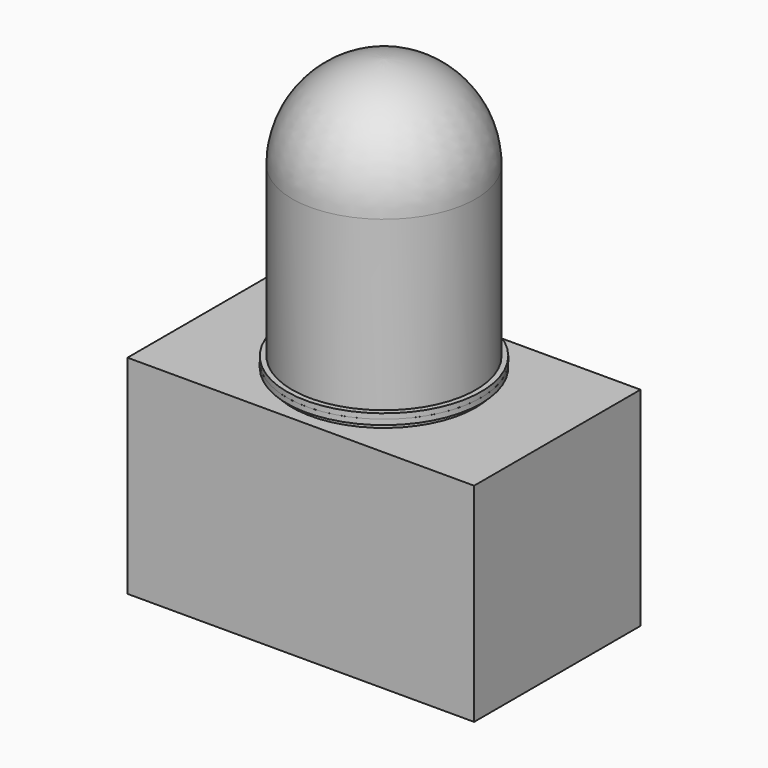
from build123d import *

# Parameters (mm, degrees)
F0_W      = 3
F0_H      = 3
F2_R      = 56
F2_R_2    = 50
F3_DEPTH  = 3
F4_R      = 53
F4_R_2    = 50
F5_DEPTH  = 3
F6_W      = 200
F6_H      = 120
F7_DEPTH  = 120
F8_T      = 3
F9_R      = 50
F10_DEPTH = 4


# Not quite as in the source:
# - a shell that OpenCascade refuses in one call is made with other operations: the cavity is built on its own and cut out


with BuildPart() as f1:
    # F0 (on Front) → F1 (revolve)
    with BuildSketch(Plane.XZ):
        with Locations((-54.5, 1.5)):
            Rectangle(F0_W, F0_H)
        Polygon((-53, 3), (-53, 0), (-50, 0), (-50, 100), (-53, 100), align=None)
        with BuildLine():
            Line((-53, 100), (-50, 100))
            ThreePointArc((-50, 100), (-35.4201251719, 135.7429342759), (0, 151.0904042125))
            Line((0, 151.0904042125), (0, 154.0904042125))
            ThreePointArc((0, 154.0904042125), (-37.5415211912, 137.8641381384), (-53, 100))
        make_face()
    revolve(axis=Axis((0, 0, 55.2105903625), (0, 0, 1)))


with BuildPart() as f3:
    # F2 (on face) → F3 (new body)
    with BuildSketch(Plane(origin=(0, 0, 0), x_dir=(1, 0, 0), z_dir=(0, 0, -1))):
        Circle(F2_R)
        Circle(F2_R_2, mode=Mode.SUBTRACT)
    extrude(amount=F3_DEPTH)

    # F4 (on face) → F5 (join)
    with BuildSketch(Plane(origin=(0, 0, -3), x_dir=(1, 0, 0), z_dir=(0, 0, -1))):
        Circle(F4_R)
        Circle(F4_R_2, mode=Mode.SUBTRACT)
    extrude(amount=F5_DEPTH)

    # F6 (on face) → F7 (join)
    with BuildSketch(Plane(origin=(0, 0, -6), x_dir=(1, 0, 0), z_dir=(0, 0, -1))):
        Rectangle(F6_W, F6_H)
    extrude(amount=F7_DEPTH)

    # F8: shell of thickness 3, made by hand


with BuildPart() as f8_core1:
    # F8_t2: copy of F3
    add(f3.part)

    # the walls: a layer under each face that stays
    f8_faces = [f8_core1.faces().sort_by_distance(p)[0] for p in [
        (0, -60, -66),
        (100, 0, -66),
        (-100, 0, -66),
        (-66.6666666667, 40, -6),
        (0, 60, -66),
        (-53, 0, -4.5),
        (-52.2666666667, 14.9333333333, -3),
        (-56, 0, -1.5),
        (-37.3333333333, 37.3333333333, 0),
        (-50, 0, -3),
        (0, 0, -6),
    ]]
    thicken(f8_faces, amount=-F8_T, mode=Mode.SUBTRACT)

    # F8_s3 → F8_t4 (revolve, cut)
    with BuildSketch(Plane.XZ):
        Polygon((53.03, -5.97), (53, -9), (50, -9), (50, -6), align=None)
    revolve(axis=Axis((0, 0, -6), (0, 0, -1)), mode=Mode.SUBTRACT)

    # F8_s5 → F8_t6 (revolve, cut)
    with BuildSketch(Plane.XZ):
        Polygon((53.03, -3.03), (50, -3), (50, 0), (53, 0), align=None)
    revolve(axis=Axis((0, 0, -3), (0, 0, -1)), mode=Mode.SUBTRACT)

    # F8_s7 → F8_t8 (revolve, cut)
    with BuildSketch(Plane.XZ):
        Polygon((49.97, -5.97), (53, -6), (53, -9), (50, -9), align=None)
    revolve(axis=Axis((0, 0, -6), (0, 0, -1)), mode=Mode.SUBTRACT)


with BuildPart() as f3_1:
    add(f3.part)

    # what is left inside the walls is the cavity
    f8_cavity = [f8_core1.part.solids().sort_by_distance(p)[0] for p in [
        (0, -56.97, -87),
    ]]
    add(f8_cavity, mode=Mode.SUBTRACT)

    # F9 (on face) → F10 (cut)
    with BuildSketch(Plane(origin=(0, 0, -9), x_dir=(1, 0, 0), z_dir=(0, 0, -1))):
        Circle(F9_R)
    extrude(amount=-F10_DEPTH, mode=Mode.SUBTRACT)


solid = Compound([f1.part, f3_1.part])
